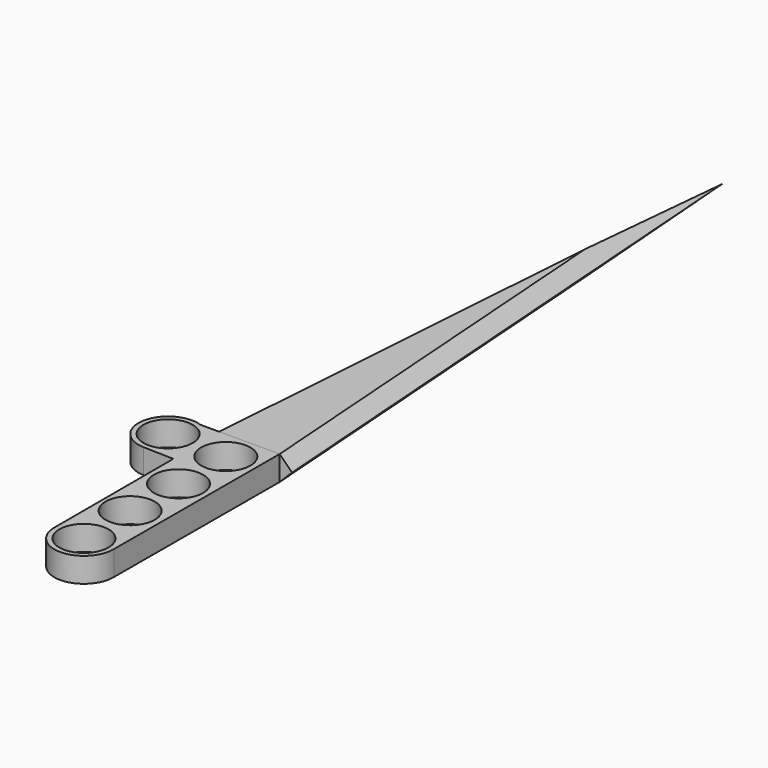
from build123d import *

# Parameters (mm, degrees)
F1_DEPTH = 3.175
F2_SIZE  = 3.17499
F3_R     = 6.35
F4_DEPTH = 6.35


# Not quite as in the source:
# - a fillet or chamfer is up to 0.001 mm smaller than in the source, because OpenCascade refuses the exact size
# - ends of sketch curves that miss each other by under 0.0002 mm in the source are joined
# - a feature names something its author has since deleted; it is built from what else it names


with BuildPart() as f1:
    # F0 (on Top) → F1 (new body, symmetric)
    with BuildSketch(Plane.XY):
        Polygon((0, 101.6), (-10.9740330666, -50.6379564073), (10.9740330666, -50.6379564073), align=None)
    extrude(amount=F1_DEPTH, both=True)

    # F2 (size 3.175 in the source; OpenCascade refuses exactly that, so slightly less here)
    f2_edges = [f1.edges().sort_by_distance(p)[0] for p in [
        (5.487017, 25.481022, 3.175),
        (-5.487017, 25.481022, 3.175),
        (5.487017, 25.481022, -3.175),
        (-5.487017, 25.481022, -3.175),
    ]]
    chamfer(f2_edges, length=F2_SIZE)


with BuildPart() as f4:
    # F3 (on face) → F4 (new body)
    with BuildSketch(Plane.XY.offset(3.175)):
        with BuildLine():
            Line((-7.6165116267, -65.6536943669), (-7.5981611835, -104.5492119633))
            ThreePointArc((-7.5981611835, -104.5492119633), (0.3625233188, -111.5840883864), (7.6185574498, -103.8244522658))
            Line((7.6185574498, -103.8244522658), (7.7907947724, -50.6379564073))
            Line((7.7907947724, -50.6379564073), (0, -50.6379564073))
            Line((0, -50.6379564073), (-7.7908047984, -50.6379564073))
            Line((-7.7908047984, -50.6379564073), (-12.6483816852, -50.6379564073))
            ThreePointArc((-12.6483816852, -50.6379564073), (-22.7193690915, -56.3837372477), (-15.4575681017, -65.4228207847))
            Line((-15.4575681017, -65.4228207847), (-7.6165116267, -65.6536943669))
        make_face()
        with Locations((-15.2333005435, -57.806121758)):
            Circle(F3_R, mode=Mode.SUBTRACT)
        with BuildLine():
            ThreePointArc((-7.6200625985, -58.1270703408), (-7.6182081929, -58.0795600348), (-7.6166502718, -58.0320390827))
            ThreePointArc((-7.6166502718, -58.0320390827), (-7.6191889591, -58.1467826471), (-7.619999152, -58.2615514324))
            Line((-7.619999152, -58.2615514324), (-7.6200625985, -58.1270703408))
        make_face(mode=Mode.SUBTRACT)
        with Locations((0, -103.9727168383)):
            Circle(F3_R, mode=Mode.SUBTRACT)
        with Locations((-0.2825671034, -88.7353366228)):
            Circle(F3_R, mode=Mode.SUBTRACT)
        with Locations((0, -73.4979564073)):
            Circle(F3_R, mode=Mode.SUBTRACT)
        with Locations((0, -58.2579564073)):
            Circle(F3_R, mode=Mode.SUBTRACT)
        with BuildLine():
            ThreePointArc((-7.619999152, -58.2615514324), (-7.6191889591, -58.1467826471), (-7.6166502718, -58.0320390827))
            ThreePointArc((-7.6166502718, -58.0320390827), (-7.6182081929, -58.0795600348), (-7.6200625985, -58.1270703408))
            Line((-7.6200625985, -58.1270703408), (-7.619999152, -58.2615514324))
        make_face()
    extrude(amount=-F4_DEPTH)


solid = Compound([f1.part, f4.part])
